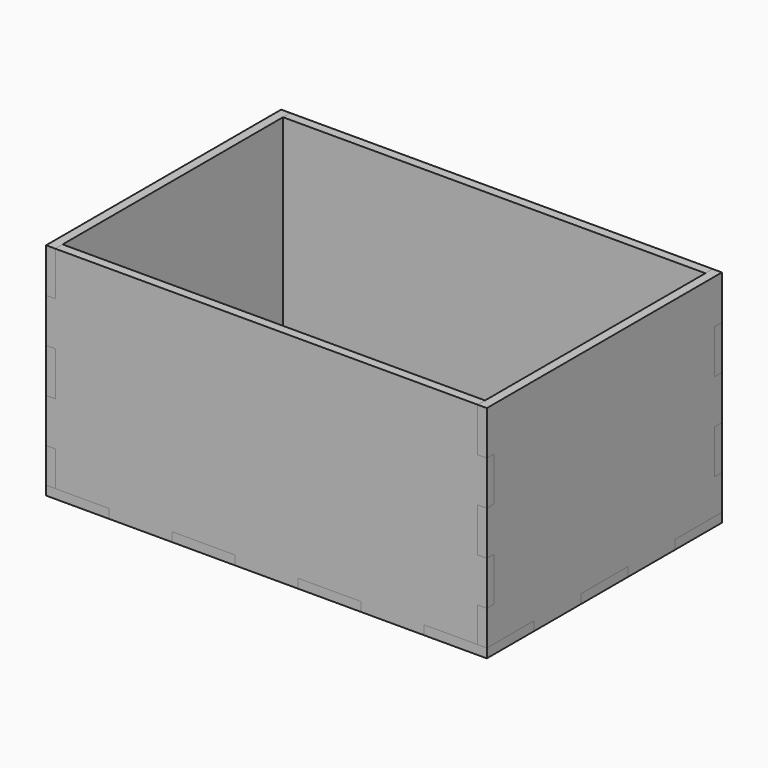
from build123d import *

# Parameters (mm, degrees)
F0_W     = 3.175
F0_H     = 3.175
F0_W_2   = 18.5964285714
F0_H_2   = 17.145
F0_H_3   = 20.32
F0_W_3   = 21.7714285714
F1_DEPTH = 3.175
F2_W     = 3.175
F2_H     = 15.24
F2_H_2   = 12.065
F2_H_3   = 3.175
F3_DEPTH = 3.175
F7_DEPTH = 3.175


with BuildPart() as f1:
    # F0 (on Top) → F1 (new body)
    with BuildSketch(Plane.XY):
        with Locations((-74.6125, 49.2125)):
            Rectangle(F0_W, F0_H)
        with Locations((-63.7267857143, 49.2125)):
            Rectangle(F0_W_2, F0_H)
        with Locations((-74.6125, 39.0525)):
            Rectangle(F0_W, F0_H_2)
        Polygon((73.025, 30.48), (73.025, 47.625), (54.4285714286, 47.625), (32.6571428571, 47.625), (10.8857142857, 47.625), (-10.8857142857, 47.625), (-32.6571428571, 47.625), (-54.4285714286, 47.625), (-73.025, 47.625), (-73.025, 30.48), (-73.025, 10.16), (-73.025, -10.16), (-73.025, -30.48), (-73.025, -47.625), (-54.4285714286, -47.625), (-32.6571428571, -47.625), (-10.8857142857, -47.625), (10.8857142857, -47.625), (32.6571428571, -47.625), (54.4285714286, -47.625), (73.025, -47.625), (73.025, -30.48), (73.025, -10.16), (73.025, 10.16), align=None)
        with Locations((-74.6125, 0)):
            Rectangle(F0_W, F0_H_3)
        with Locations((-74.6125, -39.0525)):
            Rectangle(F0_W, F0_H_2)
        with Locations((-74.6125, -49.2125)):
            Rectangle(F0_W, F0_H)
        with Locations((-63.7267857143, -49.2125)):
            Rectangle(F0_W_2, F0_H)
        with Locations((-21.7714285714, -49.2125)):
            Rectangle(F0_W_3, F0_H)
        with Locations((21.7714285714, -49.2125)):
            Rectangle(F0_W_3, F0_H)
        with Locations((63.7267857143, -49.2125)):
            Rectangle(F0_W_2, F0_H)
        with Locations((74.6125, -49.2125)):
            Rectangle(F0_W, F0_H)
        with Locations((74.6125, -39.0525)):
            Rectangle(F0_W, F0_H_2)
        with Locations((74.6125, 0)):
            Rectangle(F0_W, F0_H_3)
        with Locations((74.6125, 39.0525)):
            Rectangle(F0_W, F0_H_2)
        with Locations((74.6125, 49.2125)):
            Rectangle(F0_W, F0_H)
        with Locations((63.7267857143, 49.2125)):
            Rectangle(F0_W_2, F0_H)
        with Locations((21.7714285714, 49.2125)):
            Rectangle(F0_W_3, F0_H)
        with Locations((-21.7714285714, 49.2125)):
            Rectangle(F0_W_3, F0_H)
    extrude(amount=F1_DEPTH)


with BuildPart() as f3:
    # F2 (on face) → F3 (new body)
    with BuildSketch(Plane.YZ.offset(76.2)):
        with Locations((-49.2125, 68.58)):
            Rectangle(F2_W, F2_H)
        Polygon((-30.48, 3.175), (-30.48, 0), (47.625, 0), (47.625, 15.24), (47.625, 30.48), (47.625, 45.72), (47.625, 60.96), (47.625, 76.2), (-47.625, 76.2), (-47.625, 60.96), (-47.625, 45.72), (-47.625, 30.48), (-47.625, 15.24), (-47.625, 3.175), align=None)
        with Locations((-49.2125, 38.1)):
            Rectangle(F2_W, F2_H)
        with Locations((-49.2125, 9.2075)):
            Rectangle(F2_W, F2_H_2)
        with Locations((-49.2125, 1.5875)):
            Rectangle(F2_W, F2_H_3)
        with Locations((49.2125, 7.62)):
            Rectangle(F2_W, F2_H)
        with Locations((49.2125, 38.1)):
            Rectangle(F2_W, F2_H)
        with Locations((49.2125, 68.58)):
            Rectangle(F2_W, F2_H)
    extrude(amount=-F3_DEPTH)


with BuildPart() as f4_1:
    # F4: instance of F3
    add(f3.part.mirror(Plane.YZ))

    # F5: cut F1
    add(f1.part, mode=Mode.SUBTRACT)


with BuildPart() as f3_1:
    add(f3.part)

    # F5: cut F1
    add(f1.part, mode=Mode.SUBTRACT)


with BuildPart() as f7:
    # F6 (on face) → F7 (new body)
    with BuildSketch(Plane(origin=(0, 50.8, 0), x_dir=(-1, 0, 0), z_dir=(0, 1, 0))):
        Polygon((-54.4285714286, 3.175), (-54.4285714286, 0), (76.2, 0), (76.2, 76.2), (-76.2, 76.2), (-76.2, 3.175), align=None)
    extrude(amount=-F7_DEPTH)


with BuildPart() as f8_1:
    # F8: instance of F7
    add(f7.part.mirror(Plane.XZ))

    # F9: cut F3, F4_1, F1
    add(f3_1.part, mode=Mode.SUBTRACT)
    add(f4_1.part, mode=Mode.SUBTRACT)
    add(f1.part, mode=Mode.SUBTRACT)


with BuildPart() as f7_1:
    add(f7.part)

    # F9: cut F3, F4_1, F1
    add(f3_1.part, mode=Mode.SUBTRACT)
    add(f4_1.part, mode=Mode.SUBTRACT)
    add(f1.part, mode=Mode.SUBTRACT)


solid = Compound([f1.part, f4_1.part, f3_1.part, f8_1.part, f7_1.part])
